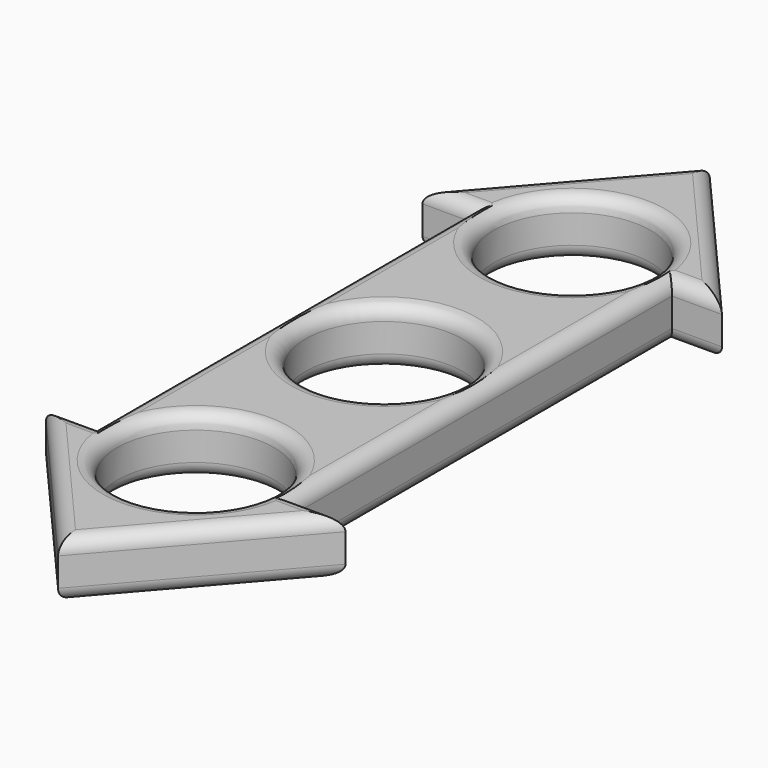
from build123d import *

# Parameters (mm, degrees)
F0_R          = 5.5
F1_DEPTH      = 4
F2_T1_DEPTH   = 33
F2_T3_DEPTH   = 6
F2_T5_DEPTH   = 21
F2_T7_DEPTH   = 21
F2_T9_DEPTH   = 6
F2_T11_DEPTH  = 21
F2_T13_DEPTH  = 21
F2_T31_DEPTH  = 8.5
F2_T35_DEPTH  = 35.5
F2_T42_DEPTH  = 8.5
F2_T46_DEPTH  = 35.5
F2_T53_DEPTH  = 35.5
F2_T57_DEPTH  = 8.5
F2_T64_DEPTH  = 8.5
F2_T68_DEPTH  = 35.5
F2_T75_DEPTH  = 8.5
F2_T79_DEPTH  = 35.5
F2_T86_DEPTH  = 35.5
F2_T90_DEPTH  = 8.5
F2_T97_DEPTH  = 8.5
F2_T101_DEPTH = 35.5
F2_T108_DEPTH = 35.5
F2_T112_DEPTH = 8.5


# Not quite as in the source:
# - a fillet or chamfer that OpenCascade refuses, or shapes differently, is made with other operations: its cross-section is extruded or revolved along the edge and cut away or added


with BuildPart() as f1:
    # F0 (on Top) → F1 (new body)
    with BuildSketch(Plane.XY):
        Polygon((-10.5, 16.5), (-7, 16.5), (-7, -16.5), (-10.5, -16.5), (0, -28.5726964676), (10.5, -16.5), (7, -16.5), (7, 16.5), (10.5, 16.5), (0, 28.5726964676), align=None)
        with BuildLine():
            ThreePointArc((5.5, -16.5), (0, -22), (-5.5, -16.5))
            ThreePointArc((-5.5, -16.5), (0, -11), (5.5, -16.5))
        make_face(mode=Mode.SUBTRACT)
        Circle(F0_R, mode=Mode.SUBTRACT)
        with BuildLine():
            ThreePointArc((5.5, 16.5), (0, 11), (-5.5, 16.5))
            ThreePointArc((-5.5, 16.5), (0, 22), (5.5, 16.5))
        make_face(mode=Mode.SUBTRACT)
    extrude(amount=F1_DEPTH)

    # F2: fillet of radius 1 on 28 edges, made by hand

    # F2_s2 → F2_t1 (cut)
    with BuildSketch(Plane.XZ.offset(-16.5)):
        with BuildLine():
            ThreePointArc((-6, 0), (-6.7071067812, 0.2928932188), (-7, 1))
            Line((-7, 1), (-7, 0))
            Line((-7, 0), (-6, 0))
        make_face()
        with BuildLine():
            ThreePointArc((7, 1), (6.7071067812, 0.2928932188), (6, 0))
            Line((6, 0), (7, 0))
            Line((7, 0), (7, 1))
        make_face()
        with BuildLine():
            ThreePointArc((-6, 4), (-6.7071067812, 3.7071067812), (-7, 3))
            Line((-7, 3), (-7, 4))
            Line((-7, 4), (-6, 4))
        make_face()
        with BuildLine():
            ThreePointArc((6, 4), (6.7071067812, 3.7071067812), (7, 3))
            Line((7, 3), (7, 4))
            Line((7, 4), (6, 4))
        make_face()
    extrude(amount=F2_T1_DEPTH, mode=Mode.SUBTRACT)

    # F2_s4 → F2_t3 (cut)
    with BuildSketch(Plane.YZ.offset(-13)):
        with BuildLine():
            ThreePointArc((16.5, 3), (16.7928932188, 3.7071067812), (17.5, 4))
            Line((17.5, 4), (16.5, 4))
            Line((16.5, 4), (16.5, 3))
        make_face()
        with BuildLine():
            ThreePointArc((-17.5, 4), (-16.7928932188, 3.7071067812), (-16.5, 3))
            Line((-16.5, 3), (-16.5, 4))
            Line((-16.5, 4), (-17.5, 4))
        make_face()
        with BuildLine():
            ThreePointArc((16.5, 1), (16.7928932188, 0.2928932188), (17.5, 0))
            Line((17.5, 0), (16.5, 0))
            Line((16.5, 0), (16.5, 1))
        make_face()
        with BuildLine():
            ThreePointArc((-16.5, 1), (-16.7928932188, 0.2928932188), (-17.5, 0))
            Line((-17.5, 0), (-16.5, 0))
            Line((-16.5, 0), (-16.5, 1))
        make_face()
    extrude(amount=F2_T3_DEPTH, mode=Mode.SUBTRACT)

    # F2_s6 → F2_t5 (cut)
    with BuildSketch(Plane(origin=(2.0076939962, -2.3084076396, 0), x_dir=(0, 0, 1), z_dir=(0.65625, -0.7545435292, 0))):
        with BuildLine():
            ThreePointArc((4, 17.7508320569), (3.7071067812, 18.4579388381), (3, 18.7508320569))
            Line((3, 18.7508320569), (4, 18.7508320569))
            Line((4, 18.7508320569), (4, 17.7508320569))
        make_face()
        with BuildLine():
            ThreePointArc((1, 18.7508320569), (0.2928932188, 18.4579388381), (0, 17.7508320569))
            Line((0, 17.7508320569), (0, 18.7508320569))
            Line((0, 18.7508320569), (1, 18.7508320569))
        make_face()
    extrude(amount=F2_T5_DEPTH, mode=Mode.SUBTRACT)

    # F2_s8 → F2_t7 (cut)
    with BuildSketch(Plane(origin=(-15.7889439962, -18.1538217534, 0), x_dir=(0, 0, 1), z_dir=(0.65625, 0.7545435292, 0))):
        with BuildLine():
            ThreePointArc((4, 17.7508320569), (3.7071067812, 18.4579388381), (3, 18.7508320569))
            Line((3, 18.7508320569), (4, 18.7508320569))
            Line((4, 18.7508320569), (4, 17.7508320569))
        make_face()
        with BuildLine():
            ThreePointArc((1, 18.7508320569), (0.2928932188, 18.4579388381), (0, 17.7508320569))
            Line((0, 17.7508320569), (0, 18.7508320569))
            Line((0, 18.7508320569), (1, 18.7508320569))
        make_face()
    extrude(amount=F2_T7_DEPTH, mode=Mode.SUBTRACT)

    # F2_s10 → F2_t9 (cut)
    with BuildSketch(Plane.YZ.offset(7)):
        with BuildLine():
            ThreePointArc((-17.5, 4), (-16.7928932188, 3.7071067812), (-16.5, 3))
            Line((-16.5, 3), (-16.5, 4))
            Line((-16.5, 4), (-17.5, 4))
        make_face()
        with BuildLine():
            ThreePointArc((17.5, 4), (16.7928932188, 3.7071067812), (16.5, 3))
            Line((16.5, 3), (16.5, 4))
            Line((16.5, 4), (17.5, 4))
        make_face()
        with BuildLine():
            ThreePointArc((-16.5, 1), (-16.7928932188, 0.2928932188), (-17.5, 0))
            Line((-17.5, 0), (-16.5, 0))
            Line((-16.5, 0), (-16.5, 1))
        make_face()
        with BuildLine():
            ThreePointArc((16.5, 1), (16.7928932188, 0.2928932188), (17.5, 0))
            Line((17.5, 0), (16.5, 0))
            Line((16.5, 0), (16.5, 1))
        make_face()
    extrude(amount=F2_T9_DEPTH, mode=Mode.SUBTRACT)

    # F2_s12 → F2_t11 (cut)
    with BuildSketch(Plane(origin=(-2.0076939962, 2.3084076396, 0), x_dir=(0, 0, 1), z_dir=(-0.65625, 0.7545435292, 0))):
        with BuildLine():
            ThreePointArc((4, 17.7508320569), (3.7071067812, 18.4579388381), (3, 18.7508320569))
            Line((3, 18.7508320569), (4, 18.7508320569))
            Line((4, 18.7508320569), (4, 17.7508320569))
        make_face()
        with BuildLine():
            ThreePointArc((1, 18.7508320569), (0.2928932188, 18.4579388381), (0, 17.7508320569))
            Line((0, 17.7508320569), (0, 18.7508320569))
            Line((0, 18.7508320569), (1, 18.7508320569))
        make_face()
    extrude(amount=F2_T11_DEPTH, mode=Mode.SUBTRACT)

    # F2_s14 → F2_t13 (cut)
    with BuildSketch(Plane(origin=(15.7889439962, 18.1538217534, 0), x_dir=(0, 0, 1), z_dir=(-0.65625, -0.7545435292, 0))):
        with BuildLine():
            ThreePointArc((4, 17.7508320569), (3.7071067812, 18.4579388381), (3, 18.7508320569))
            Line((3, 18.7508320569), (4, 18.7508320569))
            Line((4, 18.7508320569), (4, 17.7508320569))
        make_face()
        with BuildLine():
            ThreePointArc((0, 17.7508320569), (0.2928932188, 18.4579388381), (1, 18.7508320569))
            Line((1, 18.7508320569), (0, 18.7508320569))
            Line((0, 18.7508320569), (0, 17.7508320569))
        make_face()
    extrude(amount=F2_T13_DEPTH, mode=Mode.SUBTRACT)

    # F2_s15 → F2_t16 (revolve, cut)
    with BuildSketch(Plane.XZ.offset(16.5)):
        with BuildLine():
            ThreePointArc((-6.5, 4), (-5.7928932188, 3.7071067812), (-5.5, 3))
            Line((-5.5, 3), (-5.5, 4))
            Line((-5.5, 4), (-6.5, 4))
        make_face()
    revolve(axis=Axis((0, -16.5, 4), (0, 0, 1)), mode=Mode.SUBTRACT)

    # F2_s17 → F2_t18 (revolve, cut)
    with BuildSketch(Plane.XZ):
        with BuildLine():
            ThreePointArc((6.5, 4), (5.7928932188, 3.7071067812), (5.5, 3))
            Line((5.5, 3), (5.5, 4))
            Line((5.5, 4), (6.5, 4))
        make_face()
    revolve(axis=Axis((0, 0, 4), (0, 0, 1)), mode=Mode.SUBTRACT)

    # F2_s19 → F2_t20 (revolve, cut)
    with BuildSketch(Plane.XZ.offset(-16.5)):
        with BuildLine():
            ThreePointArc((-6.5, 4), (-5.7928932188, 3.7071067812), (-5.5, 3))
            Line((-5.5, 3), (-5.5, 4))
            Line((-5.5, 4), (-6.5, 4))
        make_face()
    revolve(axis=Axis((0, 16.5, 4), (0, 0, 1)), mode=Mode.SUBTRACT)

    # F2_s21 → F2_t22 (revolve, cut)
    with BuildSketch(Plane.XZ.offset(16.5)):
        with BuildLine():
            ThreePointArc((-5.5, 1), (-5.7928932188, 0.2928932188), (-6.5, 0))
            Line((-6.5, 0), (-5.5, 0))
            Line((-5.5, 0), (-5.5, 1))
        make_face()
    revolve(axis=Axis((0, -16.5, 0), (0, 0, -1)), mode=Mode.SUBTRACT)

    # F2_s23 → F2_t24 (revolve, cut)
    with BuildSketch(Plane.XZ):
        with BuildLine():
            ThreePointArc((5.5, 1), (5.7928932188, 0.2928932188), (6.5, 0))
            Line((6.5, 0), (5.5, 0))
            Line((5.5, 0), (5.5, 1))
        make_face()
    revolve(axis=Axis((0, 0, 0), (0, 0, 1)), mode=Mode.SUBTRACT)

    # F2_s25 → F2_t26 (revolve, cut)
    with BuildSketch(Plane.XZ.offset(-16.5)):
        with BuildLine():
            ThreePointArc((-5.5, 1), (-5.7928932188, 0.2928932188), (-6.5, 0))
            Line((-6.5, 0), (-5.5, 0))
            Line((-5.5, 0), (-5.5, 1))
        make_face()
    revolve(axis=Axis((0, 16.5, 0), (0, 0, -1)), mode=Mode.SUBTRACT)


with BuildPart() as f2_tool29:
    # F2_s30 → F2_t31 (new body)
    with BuildSketch(Plane.YZ.offset(-13)):
        with BuildLine():
            ThreePointArc((16.5, 1), (16.7928932188, 0.2928932188), (17.5, 0))
            Line((17.5, 0), (16.5, 0))
            Line((16.5, 0), (16.5, 1))
        make_face()
    extrude(amount=F2_T31_DEPTH)

    split(bisect_by=Plane.YZ.offset(-7), keep=Keep.TOP)


with BuildPart() as f2_tool33:
    # F2_s34 → F2_t35 (new body)
    with BuildSketch(Plane.XZ.offset(-19)):
        with BuildLine():
            ThreePointArc((-6, 0), (-6.7071067812, 0.2928932188), (-7, 1))
            Line((-7, 1), (-7, 0))
            Line((-7, 0), (-6, 0))
        make_face()
    extrude(amount=F2_T35_DEPTH)

    split(bisect_by=Plane.XZ.offset(-16.5), keep=Keep.BOTTOM)


with BuildPart() as f2_tool29_1:
    add(f2_tool29.part)

    # F2_t37: intersect F2_tool33
    add(f2_tool33.part, mode=Mode.INTERSECT)


with BuildPart() as f1_1:
    add(f1.part)

    # F2_t27: cut F2_tool29
    add(f2_tool29_1.part, mode=Mode.SUBTRACT)


with BuildPart() as f2_tool40:
    # F2_s41 → F2_t42 (new body)
    with BuildSketch(Plane.YZ.offset(-4.5)):
        with BuildLine():
            ThreePointArc((-16.5, 1), (-16.7928932188, 0.2928932188), (-17.5, 0))
            Line((-17.5, 0), (-16.5, 0))
            Line((-16.5, 0), (-16.5, 1))
        make_face()
    extrude(amount=-F2_T42_DEPTH)

    split(bisect_by=Plane.YZ.offset(-7), keep=Keep.TOP)


with BuildPart() as f2_tool44:
    # F2_s45 → F2_t46 (new body)
    with BuildSketch(Plane.XZ.offset(-16.5)):
        with BuildLine():
            ThreePointArc((-6, 0), (-6.7071067812, 0.2928932188), (-7, 1))
            Line((-7, 1), (-7, 0))
            Line((-7, 0), (-6, 0))
        make_face()
    extrude(amount=F2_T46_DEPTH)

    split(bisect_by=Plane.XZ.offset(16.5), keep=Keep.TOP)


with BuildPart() as f2_tool40_1:
    add(f2_tool40.part)

    # F2_t48: intersect F2_tool44
    add(f2_tool44.part, mode=Mode.INTERSECT)


with BuildPart() as f1_2:
    add(f1_1.part)

    # F2_t38: cut F2_tool40
    add(f2_tool40_1.part, mode=Mode.SUBTRACT)


with BuildPart() as f2_tool51:
    # F2_s52 → F2_t53 (new body)
    with BuildSketch(Plane.XZ.offset(19)):
        with BuildLine():
            ThreePointArc((7, 1), (6.7071067812, 0.2928932188), (6, 0))
            Line((6, 0), (7, 0))
            Line((7, 0), (7, 1))
        make_face()
    extrude(amount=-F2_T53_DEPTH)

    split(bisect_by=Plane.XZ.offset(16.5), keep=Keep.TOP)


with BuildPart() as f2_tool55:
    # F2_s56 → F2_t57 (new body)
    with BuildSketch(Plane.YZ.offset(13)):
        with BuildLine():
            ThreePointArc((-16.5, 1), (-16.7928932188, 0.2928932188), (-17.5, 0))
            Line((-17.5, 0), (-16.5, 0))
            Line((-16.5, 0), (-16.5, 1))
        make_face()
    extrude(amount=-F2_T57_DEPTH)

    split(bisect_by=Plane.YZ.offset(7), keep=Keep.BOTTOM)


with BuildPart() as f2_tool51_1:
    add(f2_tool51.part)

    # F2_t59: intersect F2_tool55
    add(f2_tool55.part, mode=Mode.INTERSECT)


with BuildPart() as f1_3:
    add(f1_2.part)

    # F2_t49: cut F2_tool51
    add(f2_tool51_1.part, mode=Mode.SUBTRACT)


with BuildPart() as f2_tool62:
    # F2_s63 → F2_t64 (new body)
    with BuildSketch(Plane.YZ.offset(4.5)):
        with BuildLine():
            ThreePointArc((16.5, 1), (16.7928932188, 0.2928932188), (17.5, 0))
            Line((17.5, 0), (16.5, 0))
            Line((16.5, 0), (16.5, 1))
        make_face()
    extrude(amount=F2_T64_DEPTH)

    split(bisect_by=Plane.YZ.offset(7), keep=Keep.BOTTOM)


with BuildPart() as f2_tool66:
    # F2_s67 → F2_t68 (new body)
    with BuildSketch(Plane.XZ.offset(16.5)):
        with BuildLine():
            ThreePointArc((7, 1), (6.7071067812, 0.2928932188), (6, 0))
            Line((6, 0), (7, 0))
            Line((7, 0), (7, 1))
        make_face()
    extrude(amount=-F2_T68_DEPTH)

    split(bisect_by=Plane.XZ.offset(-16.5), keep=Keep.BOTTOM)


with BuildPart() as f2_tool62_1:
    add(f2_tool62.part)

    # F2_t70: intersect F2_tool66
    add(f2_tool66.part, mode=Mode.INTERSECT)


with BuildPart() as f1_4:
    add(f1_3.part)

    # F2_t60: cut F2_tool62
    add(f2_tool62_1.part, mode=Mode.SUBTRACT)


with BuildPart() as f2_tool73:
    # F2_s74 → F2_t75 (new body)
    with BuildSketch(Plane.YZ.offset(-13)):
        with BuildLine():
            ThreePointArc((16.5, 3), (16.7928932188, 3.7071067812), (17.5, 4))
            Line((17.5, 4), (16.5, 4))
            Line((16.5, 4), (16.5, 3))
        make_face()
    extrude(amount=F2_T75_DEPTH)

    split(bisect_by=Plane.YZ.offset(-7), keep=Keep.TOP)


with BuildPart() as f2_tool77:
    # F2_s78 → F2_t79 (new body)
    with BuildSketch(Plane.XZ.offset(-19)):
        with BuildLine():
            ThreePointArc((-6, 4), (-6.7071067812, 3.7071067812), (-7, 3))
            Line((-7, 3), (-7, 4))
            Line((-7, 4), (-6, 4))
        make_face()
    extrude(amount=F2_T79_DEPTH)

    split(bisect_by=Plane.XZ.offset(-16.5), keep=Keep.BOTTOM)


with BuildPart() as f2_tool73_1:
    add(f2_tool73.part)

    # F2_t81: intersect F2_tool77
    add(f2_tool77.part, mode=Mode.INTERSECT)


with BuildPart() as f1_5:
    add(f1_4.part)

    # F2_t71: cut F2_tool73
    add(f2_tool73_1.part, mode=Mode.SUBTRACT)


with BuildPart() as f2_tool84:
    # F2_s85 → F2_t86 (new body)
    with BuildSketch(Plane.XZ.offset(-16.5)):
        with BuildLine():
            ThreePointArc((-6, 4), (-6.7071067812, 3.7071067812), (-7, 3))
            Line((-7, 3), (-7, 4))
            Line((-7, 4), (-6, 4))
        make_face()
    extrude(amount=F2_T86_DEPTH)

    split(bisect_by=Plane.XZ.offset(16.5), keep=Keep.TOP)


with BuildPart() as f2_tool88:
    # F2_s89 → F2_t90 (new body)
    with BuildSketch(Plane.YZ.offset(-4.5)):
        with BuildLine():
            ThreePointArc((-17.5, 4), (-16.7928932188, 3.7071067812), (-16.5, 3))
            Line((-16.5, 3), (-16.5, 4))
            Line((-16.5, 4), (-17.5, 4))
        make_face()
    extrude(amount=-F2_T90_DEPTH)

    split(bisect_by=Plane.YZ.offset(-7), keep=Keep.TOP)


with BuildPart() as f2_tool84_1:
    add(f2_tool84.part)

    # F2_t92: intersect F2_tool88
    add(f2_tool88.part, mode=Mode.INTERSECT)


with BuildPart() as f1_6:
    add(f1_5.part)

    # F2_t82: cut F2_tool84
    add(f2_tool84_1.part, mode=Mode.SUBTRACT)


with BuildPart() as f2_tool95:
    # F2_s96 → F2_t97 (new body)
    with BuildSketch(Plane.YZ.offset(13)):
        with BuildLine():
            ThreePointArc((-17.5, 4), (-16.7928932188, 3.7071067812), (-16.5, 3))
            Line((-16.5, 3), (-16.5, 4))
            Line((-16.5, 4), (-17.5, 4))
        make_face()
    extrude(amount=-F2_T97_DEPTH)

    split(bisect_by=Plane.YZ.offset(7), keep=Keep.BOTTOM)


with BuildPart() as f2_tool99:
    # F2_s100 → F2_t101 (new body)
    with BuildSketch(Plane.XZ.offset(19)):
        with BuildLine():
            ThreePointArc((6, 4), (6.7071067812, 3.7071067812), (7, 3))
            Line((7, 3), (7, 4))
            Line((7, 4), (6, 4))
        make_face()
    extrude(amount=-F2_T101_DEPTH)

    split(bisect_by=Plane.XZ.offset(16.5), keep=Keep.TOP)


with BuildPart() as f2_tool95_1:
    add(f2_tool95.part)

    # F2_t103: intersect F2_tool99
    add(f2_tool99.part, mode=Mode.INTERSECT)


with BuildPart() as f1_7:
    add(f1_6.part)

    # F2_t93: cut F2_tool95
    add(f2_tool95_1.part, mode=Mode.SUBTRACT)


with BuildPart() as f2_tool106:
    # F2_s107 → F2_t108 (new body)
    with BuildSketch(Plane.XZ.offset(16.5)):
        with BuildLine():
            ThreePointArc((6, 4), (6.7071067812, 3.7071067812), (7, 3))
            Line((7, 3), (7, 4))
            Line((7, 4), (6, 4))
        make_face()
    extrude(amount=-F2_T108_DEPTH)

    split(bisect_by=Plane.XZ.offset(-16.5), keep=Keep.BOTTOM)


with BuildPart() as f2_tool110:
    # F2_s111 → F2_t112 (new body)
    with BuildSketch(Plane.YZ.offset(4.5)):
        with BuildLine():
            ThreePointArc((17.5, 4), (16.7928932188, 3.7071067812), (16.5, 3))
            Line((16.5, 3), (16.5, 4))
            Line((16.5, 4), (17.5, 4))
        make_face()
    extrude(amount=F2_T112_DEPTH)

    split(bisect_by=Plane.YZ.offset(7), keep=Keep.BOTTOM)


with BuildPart() as f2_tool106_1:
    add(f2_tool106.part)

    # F2_t114: intersect F2_tool110
    add(f2_tool110.part, mode=Mode.INTERSECT)


with BuildPart() as f1_8:
    add(f1_7.part)

    # F2_t104: cut F2_tool106
    add(f2_tool106_1.part, mode=Mode.SUBTRACT)


solid = f1_8.part
